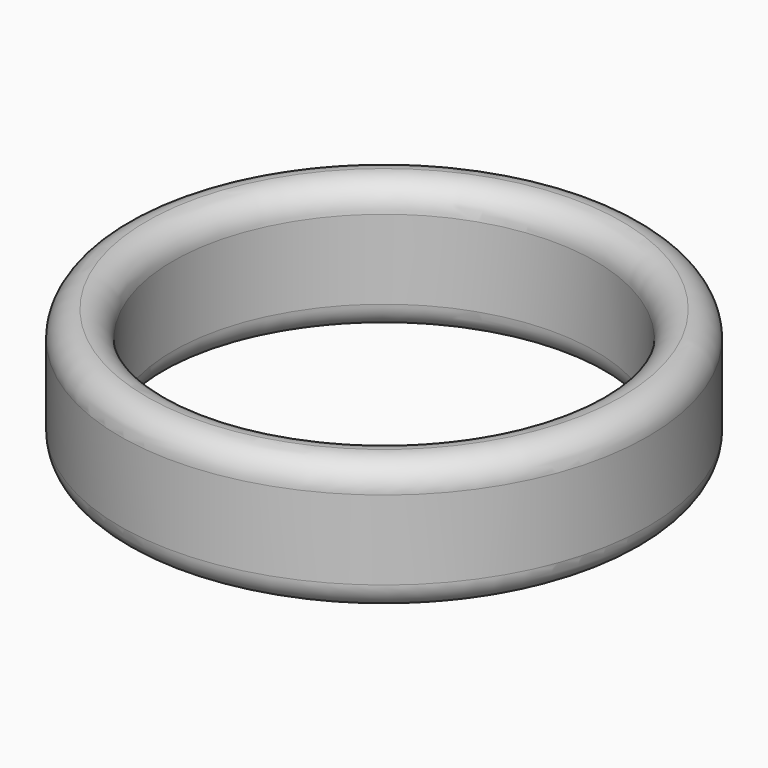
from build123d import *

# Parameters (mm, degrees)
F0_R     = 10
F0_R_2   = 8
F1_DEPTH = 5
F2_R     = 0.99999


# Not quite as in the source:
# - a fillet or chamfer is up to 0.001 mm smaller than in the source, because OpenCascade refuses the exact size


with BuildPart() as f1:
    # F0 (on Top) → F1 (new body)
    with BuildSketch(Plane.XY):
        Circle(F0_R)
        Circle(F0_R_2, mode=Mode.SUBTRACT)
    extrude(amount=F1_DEPTH)

    # F2 (radius 1 in the source; OpenCascade refuses exactly that, so slightly less here)
    f2_edges = [f1.edges().sort_by_distance(p)[0] for p in [
        (-8, 0, 5),
        (-10, 0, 5),
        (-10, 0, 0),
        (-8, 0, 0),
    ]]
    fillet(f2_edges, radius=F2_R)


solid = f1.part
